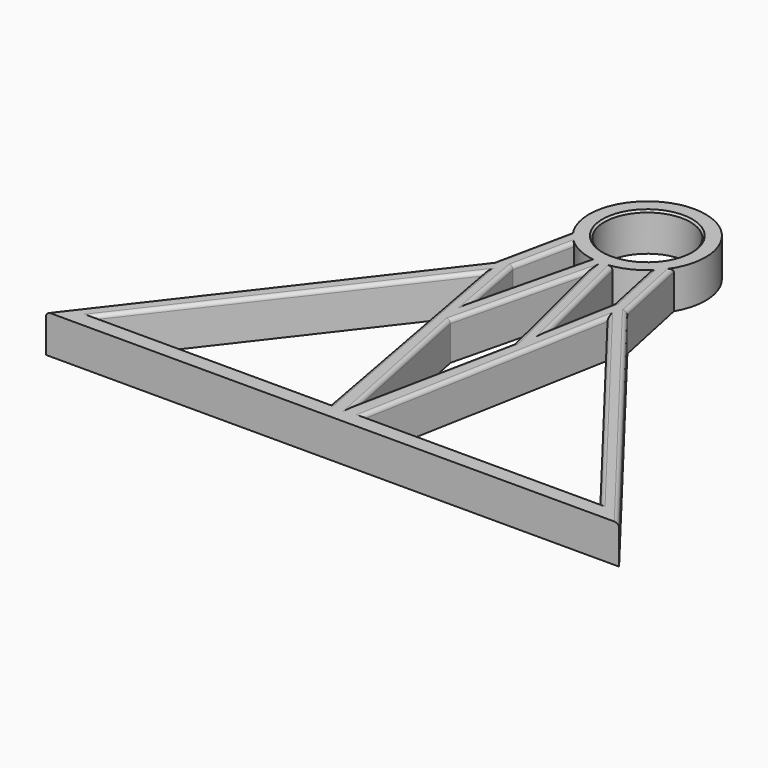
from build123d import *

# Parameters (mm, degrees)
F0_R     = 11.25
F1_DEPTH = 10
F2_DEPTH = 7.1
F3_R     = 1
F5_SIZE  = 0.5


# Not quite as in the source:
# - two fillets or chamfers of one size are made in one step
# - a feature names something its author has since deleted; it is built from what else it names


with BuildPart() as f1:
    # F0 (on Top) → F1 (new body)
    with BuildSketch(Plane.XY):
        with BuildLine():
            ThreePointArc((-2.8618452925, -14.9790634394), (0, -15.25), (2.8618452925, -14.9790634394))
            ThreePointArc((2.8618452925, -14.9790634394), (6.5768557716, -13.7589050494), (9.8594632948, -11.6341516037))
            ThreePointArc((9.8594632948, -11.6341516037), (11.6573360398, -9.8320402997), (13.1303972918, -7.7559762093))
            ThreePointArc((13.1303972918, -7.7559762093), (0, 15.25), (-13.1303972918, -7.7559762093))
            ThreePointArc((-13.1303972918, -7.7559762093), (-11.6573360398, -9.8320402997), (-9.8594632948, -11.6341516037))
            ThreePointArc((-9.8594632948, -11.6341516037), (-6.5768557716, -13.7589050494), (-2.8618452925, -14.9790634394))
        make_face()
        Circle(F0_R, mode=Mode.SUBTRACT)
        with BuildLine():
            Line((10.0593915347, -44.4443559719), (2.8618452925, -14.9790634394))
            ThreePointArc((2.8618452925, -14.9790634394), (0, -15.25), (-2.8618452925, -14.9790634394))
            Line((-2.8618452925, -14.9790634394), (-10.0593915347, -44.4443559719))
            Line((-10.0593915347, -44.4443559719), (-13.1918562915, -27.455889859))
            Line((-13.1918562915, -27.455889859), (-9.8594632948, -11.6341516037))
            ThreePointArc((-9.8594632948, -11.6341516037), (-11.6573360398, -9.8320402997), (-13.1303972918, -7.7559762093))
            Line((-13.1303972918, -7.7559762093), (-17.4770367352, -28.3932154638))
            Line((-17.4770367352, -28.3932154638), (-75, -103))
            Line((-75, -103), (75, -103))
            Line((75, -103), (17.4770367352, -28.3932154638))
            Line((17.4770367352, -28.3932154638), (13.1303972918, -7.7559762093))
            ThreePointArc((13.1303972918, -7.7559762093), (11.6573360398, -9.8320402997), (9.8594632948, -11.6341516037))
            Line((9.8594632948, -11.6341516037), (13.1918562915, -27.455889859))
            Line((13.1918562915, -27.455889859), (10.0593915347, -44.4443559719))
        make_face()
        Polygon((-66.8650551594, -99), (-16.187040587, -33.2710545609), (-4.0674293329, -99), align=None, mode=Mode.SUBTRACT)
        Polygon((66.8650551594, -99), (4.0674293329, -99), (16.187040587, -33.2710545609), align=None, mode=Mode.SUBTRACT)
        Polygon((-8.2882046257, -54.0501300567), (0, -20.1199036092), (8.2882046257, -54.0501300567), (0, -94.5818126202), align=None, mode=Mode.SUBTRACT)
    extrude(amount=F1_DEPTH)

    # F0 (on Top) → F2 (join)
    with BuildSketch(Plane.XY):
        with BuildLine():
            ThreePointArc((-2.8618452925, -14.9790634394), (0, -15.25), (2.8618452925, -14.9790634394))
            ThreePointArc((2.8618452925, -14.9790634394), (6.5768557716, -13.7589050494), (9.8594632948, -11.6341516037))
            ThreePointArc((9.8594632948, -11.6341516037), (11.6573360398, -9.8320402997), (13.1303972918, -7.7559762093))
            ThreePointArc((13.1303972918, -7.7559762093), (0, 15.25), (-13.1303972918, -7.7559762093))
            ThreePointArc((-13.1303972918, -7.7559762093), (-11.6573360398, -9.8320402997), (-9.8594632948, -11.6341516037))
            ThreePointArc((-9.8594632948, -11.6341516037), (-6.5768557716, -13.7589050494), (-2.8618452925, -14.9790634394))
        make_face()
        Circle(F0_R, mode=Mode.SUBTRACT)
    extrude(amount=F2_DEPTH)

    # F3
    f3_edges = [f1.edges().sort_by_distance(p)[0] for p in [
        (-15.303717, -18.074596, 10),
        (-11.52566, -19.545021, 10),
        (-11.625624, -35.950123, 10),
        (-46.238518, -65.696608, 10),
        (-41.526048, -66.135527, 10),
        (-10.127235, -66.135527, 10),
        (-6.460618, -29.71171, 10),
        (6.460618, -29.71171, 10),
        (11.52566, -19.545021, 10),
        (11.625624, -35.950123, 10),
        (15.303717, -18.074596, 10),
        (46.238518, -65.696608, 10),
        (41.526048, -66.135527, 10),
        (10.127235, -66.135527, 10),
        (-4.144102, -37.085017, 10),
        (-4.144102, -74.315971, 10),
        (4.144102, -74.315971, 10),
        (4.144102, -37.085017, 10),
    ]]
    fillet(f3_edges, radius=F3_R)

    # F5
    f5_edges = [f1.edges().sort_by_distance(p)[0] for p in [
        (-11.25, 0, 10),
    ]]
    chamfer(f5_edges, length=F5_SIZE)


solid = f1.part
